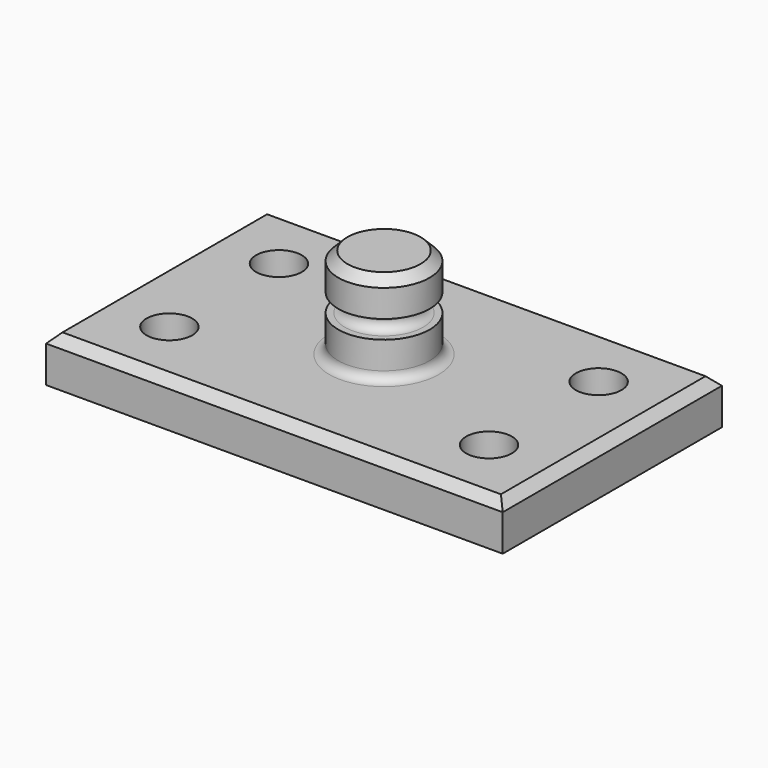
from build123d import *

# Parameters (mm, degrees)
F0_W     = 127
F0_H     = 76.2
F1_DEPTH = 12.7
F2_R     = 6.35
F3_DEPTH = 12.701
F4_SIZE  = 2.54
F7_R     = 2.53999
F8_SIZE  = 2.54


# Not quite as in the source:
# - a fillet or chamfer is up to 0.001 mm smaller than in the source, because OpenCascade refuses the exact size


with BuildPart() as f1:
    # F0 (on Top) → F1 (new body)
    with BuildSketch(Plane.XY):
        Rectangle(F0_W, F0_H)
    extrude(amount=F1_DEPTH)

    # F2 (on face) → F3 (cut, through all)
    with BuildSketch(Plane.XY.offset(12.7)):
        with Locations((-44.45, 19.05)):
            Circle(F2_R)
        with Locations((44.45, 19.05)):
            Circle(F2_R)
        with Locations((44.45, -19.05)):
            Circle(F2_R)
        with Locations((-44.45, -19.05)):
            Circle(F2_R)
    extrude(amount=-F3_DEPTH, mode=Mode.SUBTRACT)

    # F4
    f4_edges = [f1.edges().sort_by_distance(p)[0] for p in [
        (-63.5, 0, 12.7),
        (0, 38.1, 12.7),
        (0, -38.1, 12.7),
        (63.5, 0, 12.7),
    ]]
    chamfer(f4_edges, length=F4_SIZE)

    # F5 (on Front) → F6 (revolve)
    with BuildSketch(Plane.XZ):
        Polygon((0, 38.1), (0, 12.7), (12.7, 12.7), (12.7, 22.86), (8.3547569811, 22.86), (8.3547569811, 27.94), (12.7, 27.94), (12.7, 38.1), align=None)
    revolve(axis=Axis((0, 0, 25.4), (0, 0, 1)))

    # F7 (radius 2.54 in the source; OpenCascade refuses exactly that, so slightly less here)
    f7_edges = [f1.edges().sort_by_distance(p)[0] for p in [
        (-12.7, 0, 12.7),
        (-8.354757, 0, 22.86),
        (-8.354757, 0, 27.94),
    ]]
    fillet(f7_edges, radius=F7_R)

    # F8
    f8_edges = [f1.edges().sort_by_distance(p)[0] for p in [
        (-12.7, 0, 38.1),
    ]]
    chamfer(f8_edges, length=F8_SIZE)


solid = f1.part
